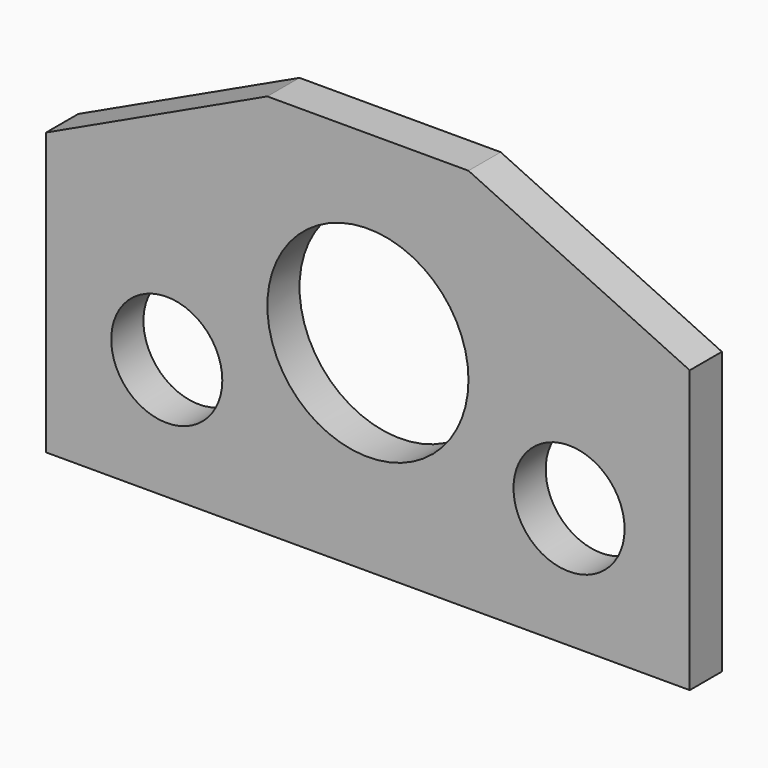
from build123d import *

# Parameters (mm, degrees)
F1_DEPTH = 6.35
F2_R     = 15.875
F2_R_2   = 8.7674107973
F3_DEPTH = 6.35


# Not quite as in the source:
# - a feature names something its author has since deleted; it is built from what else it names


with BuildPart() as f1:
    # F0 (on Front) → F1 (new body)
    with BuildSketch(Plane.XZ):
        Polygon((-15.875, 25.1552741975), (-50.8, 8.7795666171), (-50.8, -35.6704333829), (0, -35.6704333829), (0, 25.1552741975), align=None)
        Polygon((0, 25.1552741975), (0, -35.6704333829), (50.8, -35.6704333829), (50.8, 8.7795666171), (15.875, 25.1552741975), align=None)
    extrude(amount=F1_DEPTH)

    # F2 (on face) → F3 (cut)
    with BuildSketch(Plane.XZ.offset(6.35)):
        with Locations((0, -3.9204333829)):
            Circle(F2_R)
        with Locations((31.75, -16.6204333829)):
            Circle(F2_R_2)
        with Locations((-31.75, -16.6204333829)):
            Circle(F2_R_2)
    extrude(amount=-F3_DEPTH, mode=Mode.SUBTRACT)


solid = f1.part
